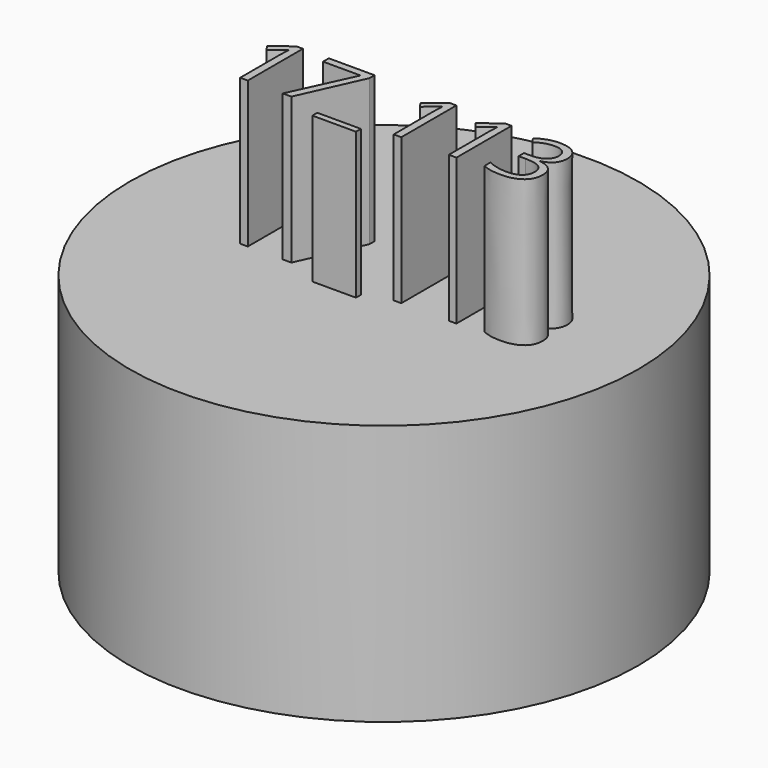
from build123d import *

# Parameters (mm, degrees)
F0_R         = 63.6489708407
F1_DEPTH     = 65.278
F2_TEXT_SIZE = 24.1359210728
F3_DEPTH     = 36.576


# Not quite as in the source:
# - Text() gives the source's letters only with a copy of the font that has no kerning and outlines rounded to 1/6400 em; it was checked with that copy


with BuildPart() as f1:
    # F0 (on Top) → F1 (new body)
    with BuildSketch(Plane.XY):
        Circle(F0_R)
    extrude(amount=F1_DEPTH)

    # F2 (on face) → F3 (join)
    with BuildSketch(Plane.XY.offset(65.278)):
        with Locations((-36.8475094438, -7.079873234)):
            Text('17_113', F2_TEXT_SIZE, font='Open Sans', text_align=(TextAlign.LEFT, TextAlign.BOTTOM))
    extrude(amount=F3_DEPTH)


solid = f1.part
